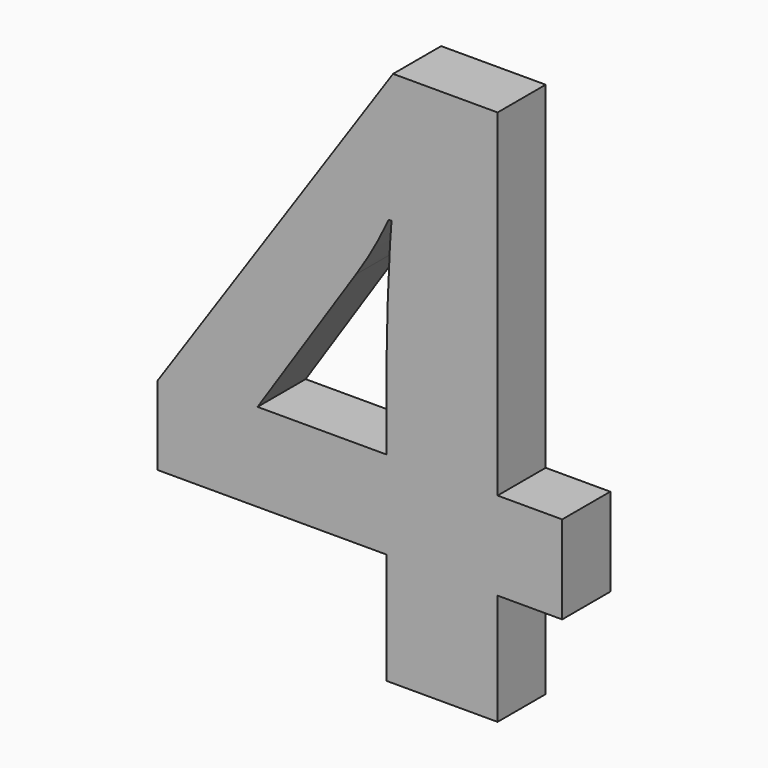
from build123d import *

# Parameters (mm, degrees)
F0_TEXT_SIZE = 62.5
F1_DEPTH     = 5


# Not quite as in the source:
# - Text() gives the source's letters only with a copy of the font that has no kerning and outlines rounded to 1/6400 em; it was checked with that copy


with BuildPart() as f1:
    # F0 (on Front) → F1 (new body)
    with BuildSketch(Plane.XZ):
        with Locations((-58.6910341797, 14.5400938902)):
            Text('4', F0_TEXT_SIZE, font='Open Sans', font_style=FontStyle.BOLD, text_align=(TextAlign.LEFT, TextAlign.BOTTOM))
    extrude(amount=F1_DEPTH)


solid = f1.part
